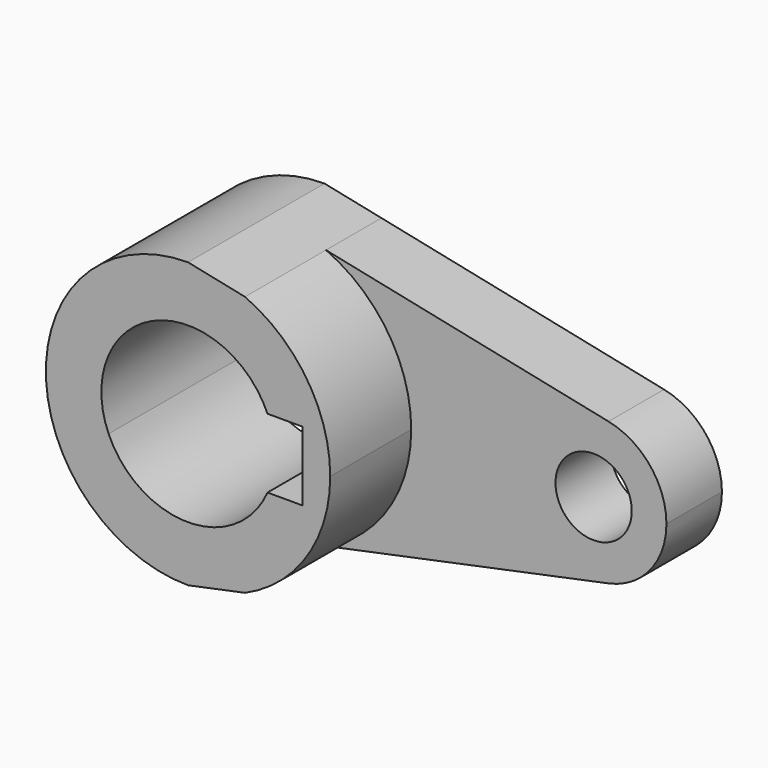
from build123d import *

# Parameters (mm, degrees)
F0_R     = 13.97
F1_DEPTH = 25.4
F2_DEPTH = 62.484


with BuildPart() as f1:
    # F0 (on Front) → F1 (new body)
    with BuildSketch(Plane.XZ):
        with BuildLine():
            Line((20.8402394137, 47.7175997005), (0, 52.07))
            ThreePointArc((0, 52.07), (-52.07, 0), (0, -52.07))
            Line((0, -52.07), (20.8402394137, -47.7175997005))
            ThreePointArc((20.8402394137, -47.7175997005), (43.5685446525, -28.5143265196), (52.07, 0))
            ThreePointArc((52.07, 0), (43.5685446525, 28.5143265196), (20.8402394137, 47.7175997005))
        make_face()
        with BuildLine():
            ThreePointArc((-29.099355663, 12.7), (0, 31.75), (29.099355663, 12.7))
            Line((29.099355663, 12.7), (41.91, 12.7))
            Line((41.91, 12.7), (41.91, -12.7))
            Line((41.91, -12.7), (29.099355663, -12.7))
            ThreePointArc((29.099355663, -12.7), (0, -31.75), (-29.099355663, -12.7))
            Line((-29.099355663, -12.7), (-41.91, -12.7))
            Line((-41.91, -12.7), (-41.91, 12.7))
            Line((-41.91, 12.7), (-29.099355663, 12.7))
        make_face(mode=Mode.SUBTRACT)
        with BuildLine():
            Line((124.3177732028, 26.1067323726), (20.8402394137, 47.7175997005))
            ThreePointArc((20.8402394137, 47.7175997005), (43.5685446525, 28.5143265196), (52.07, 0))
            ThreePointArc((52.07, 0), (43.5685446525, -28.5143265196), (20.8402394137, -47.7175997005))
            Line((20.8402394137, -47.7175997005), (124.3177732028, -26.1067323726))
            ThreePointArc((124.3177732028, -26.1067323726), (92.1954870011, 0), (124.3177732028, 26.1067323726))
        make_face()
        with BuildLine():
            ThreePointArc((145.5354870011, 0), (139.5621216671, 16.8207673279), (124.3177732028, 26.1067323726))
            ThreePointArc((124.3177732028, 26.1067323726), (92.1954870011, 0), (124.3177732028, -26.1067323726))
            ThreePointArc((124.3177732028, -26.1067323726), (139.5621216671, -16.8207673279), (145.5354870011, 0))
        make_face()
        with Locations((118.8654870011, 0)):
            Circle(F0_R, mode=Mode.SUBTRACT)
        with BuildLine():
            ThreePointArc((-29.099355663, -12.7), (-31.75, 0), (-29.099355663, 12.7))
            Line((-29.099355663, 12.7), (-41.91, 12.7))
            Line((-41.91, 12.7), (-41.91, -12.7))
            Line((-41.91, -12.7), (-29.099355663, -12.7))
        make_face()
    extrude(amount=F1_DEPTH)

    # F0 (on Front) → F2 (join)
    with BuildSketch(Plane.XZ):
        with BuildLine():
            Line((20.8402394137, 47.7175997005), (0, 52.07))
            ThreePointArc((0, 52.07), (-52.07, 0), (0, -52.07))
            Line((0, -52.07), (20.8402394137, -47.7175997005))
            ThreePointArc((20.8402394137, -47.7175997005), (43.5685446525, -28.5143265196), (52.07, 0))
            ThreePointArc((52.07, 0), (43.5685446525, 28.5143265196), (20.8402394137, 47.7175997005))
        make_face()
        with BuildLine():
            ThreePointArc((-29.099355663, 12.7), (0, 31.75), (29.099355663, 12.7))
            Line((29.099355663, 12.7), (41.91, 12.7))
            Line((41.91, 12.7), (41.91, -12.7))
            Line((41.91, -12.7), (29.099355663, -12.7))
            ThreePointArc((29.099355663, -12.7), (0, -31.75), (-29.099355663, -12.7))
            Line((-29.099355663, -12.7), (-41.91, -12.7))
            Line((-41.91, -12.7), (-41.91, 12.7))
            Line((-41.91, 12.7), (-29.099355663, 12.7))
        make_face(mode=Mode.SUBTRACT)
        with BuildLine():
            ThreePointArc((-29.099355663, -12.7), (-31.75, 0), (-29.099355663, 12.7))
            Line((-29.099355663, 12.7), (-41.91, 12.7))
            Line((-41.91, 12.7), (-41.91, -12.7))
            Line((-41.91, -12.7), (-29.099355663, -12.7))
        make_face()
    extrude(amount=F2_DEPTH)


solid = f1.part
